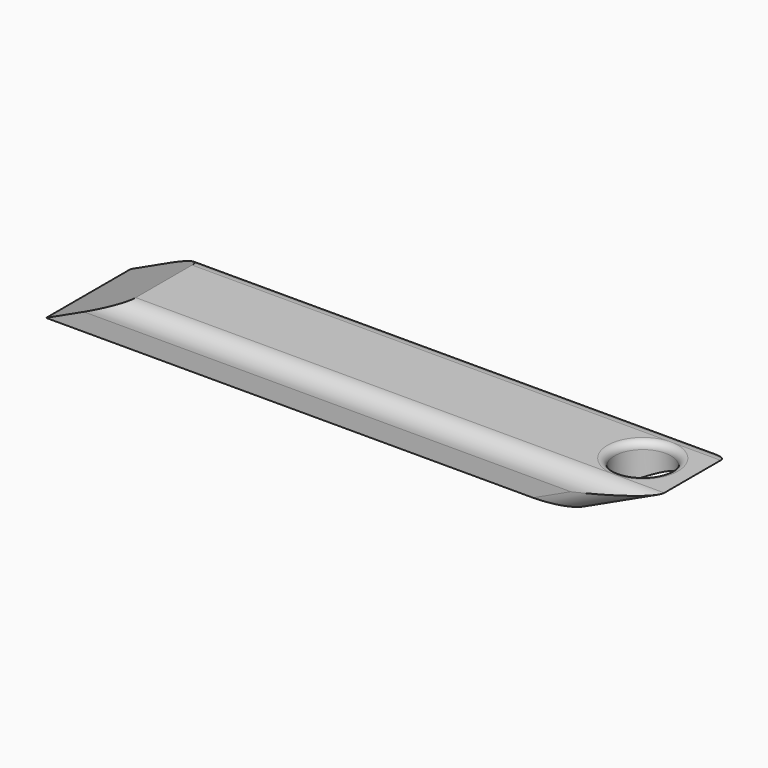
from build123d import *

# Parameters (mm, degrees)
F1_DEPTH = 30
F2_R     = 8
F3_DEPTH = 25
F4_R     = 5
F5_R     = 1.99999


# Not quite as in the source:
# - a fillet or chamfer is up to 0.001 mm smaller than in the source, because OpenCascade refuses the exact size


with BuildPart() as f1:
    # F0 (on Front) → F1 (new body)
    with BuildSketch(Plane.XZ):
        Polygon((-44.6024514475, 10), (-66.0475206525, 0), (83.9524793475, 0), (105.3975485525, 10), align=None)
    extrude(amount=F1_DEPTH)

    # F2 (on Top) → F3 (cut)
    with BuildSketch(Plane.XY):
        with Locations((91.2811756134, -15)):
            Circle(F2_R)
    extrude(amount=F3_DEPTH, mode=Mode.SUBTRACT)

    # F4
    f4_edges = [f1.edges().sort_by_distance(p)[0] for p in [
        (30.397549, 0, 10),
        (30.397549, -30, 10),
        (94.675014, -30, 5),
        (94.675014, 0, 5),
    ]]
    fillet(f4_edges, radius=F4_R)

    # F5 (radius 2 in the source; OpenCascade refuses exactly that, so slightly less here)
    f5_edges = [f1.edges().sort_by_distance(p)[0] for p in [
        (83.281176, -15, 10),
    ]]
    fillet(f5_edges, radius=F5_R)


solid = f1.part
